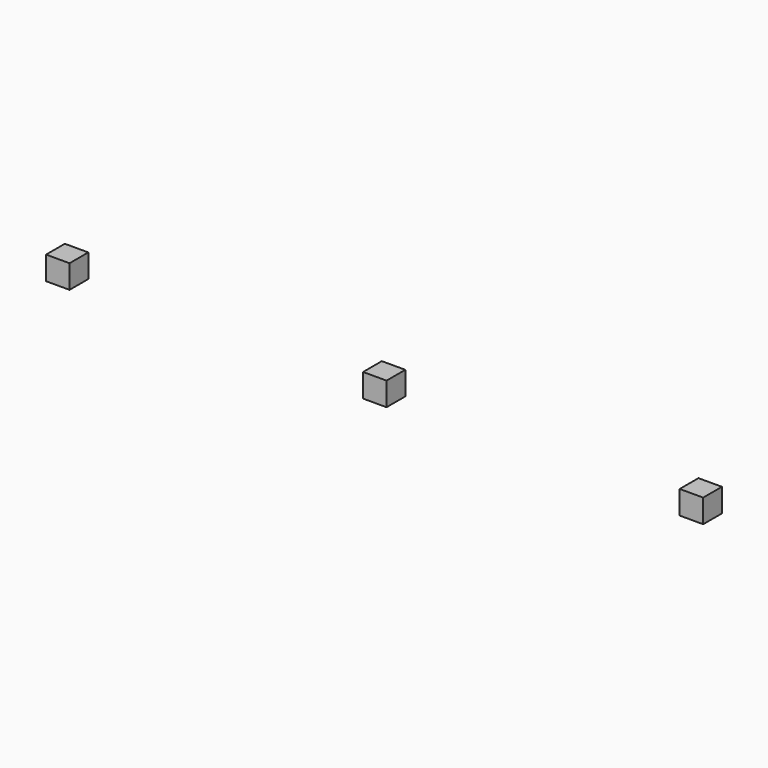
from build123d import *

# Parameters (mm, degrees)
F0_W     = 2.54
F0_H     = 2.54
F1_DEPTH = 2.54
F2_W     = 2.54
F2_H     = 2.54
F3_DEPTH = 2.54
F4_W     = 2.54
F4_H     = 2.54
F5_DEPTH = 2.54


# Not quite as in the source:
# - the program builds the solid bodies; features that only make, move or delete a surface that nothing else refers to are left out


with BuildPart() as f1:
    # F0 (on Top) → F1 (new body)
    with BuildSketch(Plane.XY):
        with Locations((0.3397457767, 0.3430546279)):
            Rectangle(F0_W, F0_H)
    extrude(amount=F1_DEPTH)


with BuildPart() as f3:
    # F2 (on Top) → F3 (new body)
    with BuildSketch(Plane.XY):
        with Locations((34.6974694668, 0.3033101014)):
            Rectangle(F2_W, F2_H)
    extrude(amount=F3_DEPTH)


with BuildPart() as f5:
    # F4 (on Top) → F5 (new body)
    with BuildSketch(Plane.XY):
        with Locations((68.9874694668, 0.2991668801)):
            Rectangle(F4_W, F4_H)
    extrude(amount=F5_DEPTH)


solid = Compound([f1.part, f3.part, f5.part])
